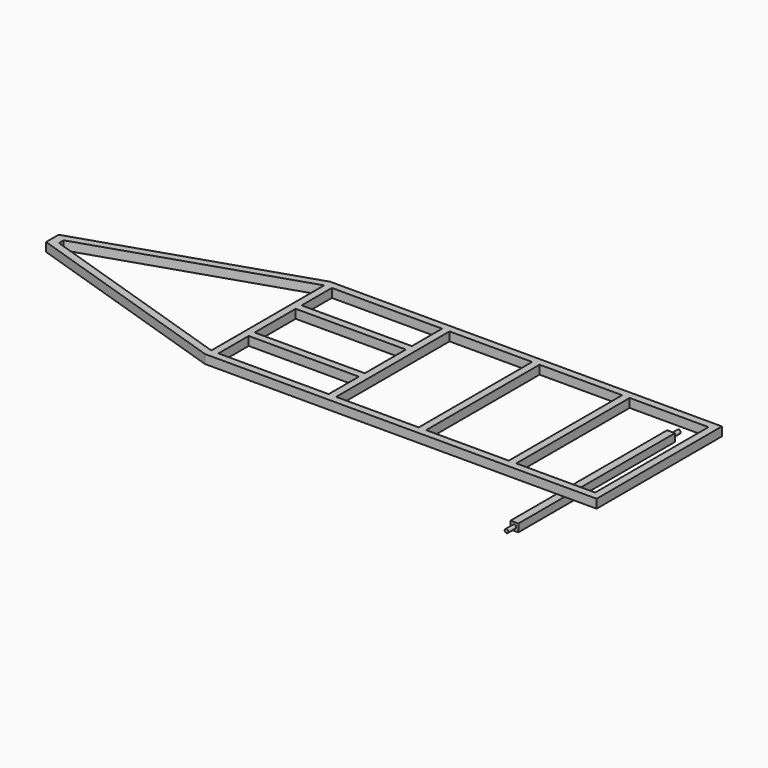
from build123d import *

# Parameters (mm, degrees)
F0_W     = 563.0000123978
F0_H     = 193
F0_H_2   = 262
F0_W_2   = 422
F0_H_3   = 724
F0_W_3   = 403
F1_DEPTH = 45
F2_W     = 40
F2_H     = 40
F2_R     = 9.4363088756
F3_DEPTH = 500
F4_DEPTH = 550


# Not quite as in the source:
# - ends of sketch curves that miss each other by under 0.0002 mm in the source are joined


with BuildPart() as f1:
    # F0 (on Top) → F1 (new body)
    with BuildSketch(Plane.XY):
        Polygon((1000, -400), (1000, 400), (-1000, 400), (-2100, 40), (-2100, -40), (-1000, -400), align=None)
        with Locations((-680.4999938011, -265.5)):
            Rectangle(F0_W, F0_H, mode=Mode.SUBTRACT)
        Polygon((-2054.0382862091, 15.0587296583), (-1000, 360.0167142359), (-1000, -360.0167142359), (-2054.0382862091, -15.0587296583), align=None, mode=Mode.SUBTRACT)
        with Locations((-680.4999938011, 0)):
            Rectangle(F0_W, F0_H_2, mode=Mode.SUBTRACT)
        with Locations((-680.4999938011, 265.5)):
            Rectangle(F0_W, F0_H, mode=Mode.SUBTRACT)
        Polygon((-361, -362), (-361, 362), (61, 362.0000114441), (61, -362), align=None, mode=Mode.SUBTRACT)
        with Locations((310, 0)):
            Rectangle(F0_W_2, F0_H_3, mode=Mode.SUBTRACT)
        with Locations((760.5, 0)):
            Rectangle(F0_W_3, F0_H_3, mode=Mode.SUBTRACT)
    extrude(amount=F1_DEPTH)


with BuildPart() as f3:
    # F2 (on Front) → F3 (new body, symmetric)
    with BuildSketch(Plane.XZ):
        with Locations((660, -150)):
            Rectangle(F2_W, F2_H)
        with Locations((660, -150)):
            Circle(F2_R, mode=Mode.SUBTRACT)
    extrude(amount=F3_DEPTH, both=True)

    # F2 (on Front) → F4 (join, symmetric)
    with BuildSketch(Plane.XZ):
        with Locations((660, -150)):
            Circle(F2_R)
    extrude(amount=F4_DEPTH, both=True)


solid = Compound([f1.part, f3.part])
